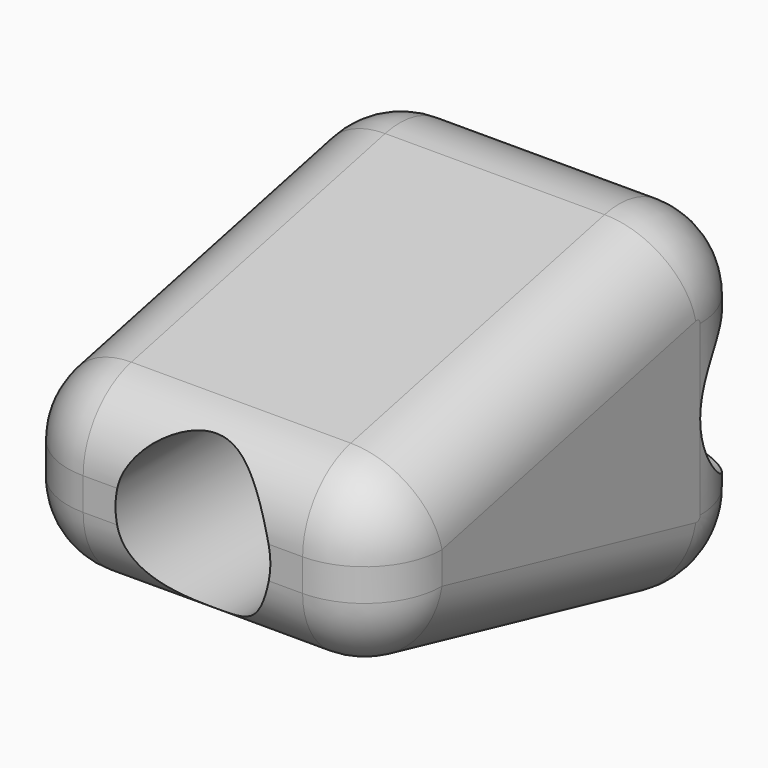
from build123d import *

# Parameters (mm, degrees)
F2_DEPTH = 14.5
F4_DEPTH = 29.001
F5_R     = 5.99999
F0_R     = 6
F6_DEPTH = 87.122


# Not quite as in the source:
# - a fillet or chamfer is up to 0.001 mm smaller than in the source, because OpenCascade refuses the exact size


with BuildPart() as f2:
    # F1 (on Right) → F2 (new body, symmetric)
    with BuildSketch(Plane.YZ):
        with BuildLine():
            Line((29.2391964545, 12.7315542681), (0, 6.0688508675))
            Line((0, 6.0688508675), (0, -5.9945774265))
            Line((0, -5.9945774265), (29.2273893105, -12.7132611239))
            ThreePointArc((29.2273893105, -12.7132611239), (34.6053079603, -11.4923680491), (37, -6.524668487))
            Line((37, -6.524668487), (37, 6.5402593021))
            ThreePointArc((37, 6.5402593021), (34.610044033, 11.5041842871), (29.2391964545, 12.7315542681))
        make_face()
    extrude(amount=F2_DEPTH, both=True)

    # F3 (on face) → F4 (cut, through all)
    with BuildSketch(Plane.YZ.offset(14.5)):
        with BuildLine():
            Line((37, -5.9922045925), (37, 6.0077954075))
            ThreePointArc((37, 6.0077954075), (31, 0.0077954075), (37, -5.9922045925))
        make_face()
    extrude(amount=-F4_DEPTH, mode=Mode.SUBTRACT)

    # F5 (radius 6 in the source; OpenCascade refuses exactly that, so slightly less here)
    f5_edges = [f2.edges().sort_by_distance(p)[0] for p in [
        (14.5, 14.619598, 9.400203),
        (14.5, 14.613695, -9.353919),
        (0, 37, 6.540259),
        (-14.5, 14.619598, 9.400203),
        (-14.5, 14.613695, -9.353919),
        (0, 0, -5.994577),
        (0, 0, 6.068851),
        (14.5, 0, 0.037137),
        (-14.5, 0, 0.037137),
    ]]
    fillet(f5_edges, radius=F5_R)

    # F0 (on Front) → F6 (cut)
    with BuildSketch(Plane.XZ):
        Circle(F0_R)
    extrude(amount=-F6_DEPTH, mode=Mode.SUBTRACT)


solid = f2.part
